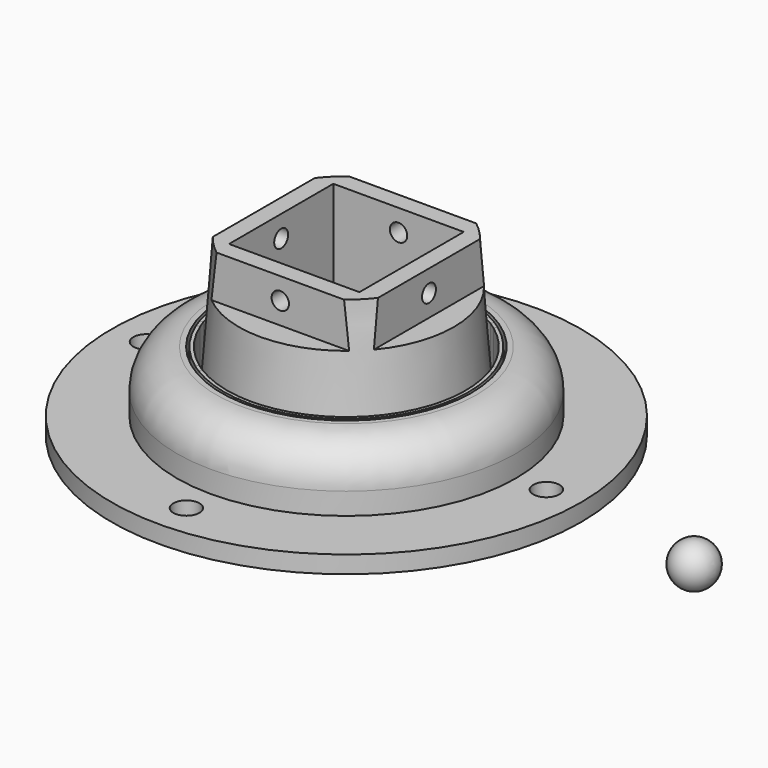
from build123d import *
from build123d import SkipClean  # not in build123d's __all__

# Parameters (mm, degrees)
F3_W           = 38.1
F3_H           = 38.1
F4_DEPTH       = 56.135
F5_DEPTH       = 12.7
F6_R           = 3.81
F7_DEPTH       = 10.415
F14_DEPTH      = 22.86
F15_R          = 6.35
F16_DEPTH      = 101.3661944055
F17_COUNT      = 10
F18_R          = 2.54
F19_DEPTH      = 68.581
F19_DEPTH_BACK = 68.581
F20_R          = 2.54
F21_DEPTH      = 107.951
F21_DEPTH_BACK = 68.581


with BuildPart() as f1:
    # F0 (on Front) → F1 (revolve)
    with BuildSketch(Plane.XZ):
        with BuildLine():
            Line((38.1, 4.445), (38.1, 0))
            Line((38.1, 0), (49.53, 0))
            Line((49.53, 0), (68.58, 0))
            Line((68.58, 0), (68.58, 5.08))
            Line((68.58, 5.08), (49.53, 5.08))
            Line((49.53, 5.08), (49.53, 11.43))
            ThreePointArc((49.53, 11.43), (46.182230509, 19.512230509), (38.1, 22.86))
            Line((38.1, 22.86), (38.1, 18.415))
            ThreePointArc((38.1, 18.415), (43.0391408666, 16.3691408666), (45.085, 11.43))
            ThreePointArc((45.085, 11.43), (43.0391408666, 6.4908591334), (38.1, 4.445))
        make_face()
        with BuildLine():
            Line((36.576, 0), (38.1, 0))
            Line((38.1, 0), (38.1, 4.445))
            ThreePointArc((38.1, 4.445), (37.3333686161, 4.4871978769), (36.576, 4.6132816546))
            Line((36.576, 4.6132816546), (36.576, 0))
        make_face()
        with BuildLine():
            ThreePointArc((36.576, 18.2467183454), (37.3333686161, 18.3728021231), (38.1, 18.415))
            Line((38.1, 18.415), (38.1, 22.86))
            Line((38.1, 22.86), (36.576, 22.86))
            Line((36.576, 22.86), (36.576, 18.2467183454))
        make_face()
    revolve(axis=Axis((0, 0, 43.4834131303), (0, 0, 1)))

    # F6 (on face) → F7 (cut, through all)
    with BuildSketch(Plane.XY.offset(5.08)):
        with Locations((0, 58.42)):
            Circle(F6_R)
        with Locations((58.42, 0)):
            Circle(F6_R)
        with Locations((0, -58.42)):
            Circle(F6_R)
        with Locations((-58.42, 0)):
            Circle(F6_R)
    extrude(amount=-F7_DEPTH, mode=Mode.SUBTRACT)


with BuildPart() as f2:
    # F0 (on Front) → F2 (revolve)
    with BuildSketch(Plane.XZ):
        with BuildLine():
            Line((34.29, 0), (34.29, 5.5755892696))
            ThreePointArc((34.29, 5.5755892696), (31.1641540477, 10.6027963216), (33.02, 16.2241448664))
            Line((33.02, 16.2241448664), (30.48, 50.8))
            Line((30.48, 50.8), (0, 50.8))
            Line((0, 50.8), (0, 0))
            Line((0, 0), (34.29, 0))
        make_face()
        Polygon((34.29, -0.254), (34.29, 0), (0, 0), (0, -5.334), (49.53, -5.334), (49.53, -0.254), align=None)
    revolve(axis=Axis((0, 0, 43.4834131303), (0, 0, 1)))

    # F3 (on face) → F4 (cut, through all)
    with BuildSketch(Plane.XY.offset(50.8)):
        Rectangle(F3_W, F3_H)
    extrude(amount=-F4_DEPTH, mode=Mode.SUBTRACT)

    # F3 (on face) → F5 (cut)
    with BuildSketch(Plane.XY.offset(50.8)):
        with BuildLine():
            Line((18.6218554392, 24.13), (22.5402639736, 24.13))
            ThreePointArc((22.5402639736, 24.13), (0, 33.02), (-22.5402639736, 24.13))
            Line((-22.5402639736, 24.13), (-18.6218554392, 24.13))
            ThreePointArc((-18.6218554392, 24.13), (0, 30.48), (18.6218554392, 24.13))
        make_face()
        with BuildLine():
            ThreePointArc((24.13, -22.5402639736), (30.717202021, -12.115027858), (33.02, 0))
            ThreePointArc((33.02, 0), (30.717202021, 12.115027858), (24.13, 22.5402639736))
            Line((24.13, 22.5402639736), (24.13, 18.6218554392))
            ThreePointArc((24.13, 18.6218554392), (28.8488543967, 9.8373776994), (30.48, 0))
            ThreePointArc((30.48, 0), (28.8488543967, -9.8373776994), (24.13, -18.6218554392))
            Line((24.13, -18.6218554392), (24.13, -22.5402639736))
        make_face()
        with BuildLine():
            ThreePointArc((-22.5402639736, -24.13), (0, -33.02), (22.5402639736, -24.13))
            Line((22.5402639736, -24.13), (18.6218554392, -24.13))
            ThreePointArc((18.6218554392, -24.13), (0, -30.48), (-18.6218554392, -24.13))
            Line((-18.6218554392, -24.13), (-22.5402639736, -24.13))
        make_face()
        with BuildLine():
            Line((-24.13, 18.6218554392), (-24.13, 22.5402639736))
            ThreePointArc((-24.13, 22.5402639736), (-33.02, 0), (-24.13, -22.5402639736))
            Line((-24.13, -22.5402639736), (-24.13, -18.6218554392))
            ThreePointArc((-24.13, -18.6218554392), (-30.48, 0), (-24.13, 18.6218554392))
        make_face()
        with BuildLine():
            Line((-18.6218554392, 24.13), (18.6218554392, 24.13))
            ThreePointArc((18.6218554392, 24.13), (0, 30.48), (-18.6218554392, 24.13))
        make_face()
        with BuildLine():
            ThreePointArc((30.48, 0), (28.8488543967, 9.8373776994), (24.13, 18.6218554392))
            Line((24.13, 18.6218554392), (24.13, -18.6218554392))
            ThreePointArc((24.13, -18.6218554392), (28.8488543967, -9.8373776994), (30.48, 0))
        make_face()
        with BuildLine():
            ThreePointArc((-18.6218554392, -24.13), (0, -30.48), (18.6218554392, -24.13))
            Line((18.6218554392, -24.13), (-18.6218554392, -24.13))
        make_face()
        with BuildLine():
            Line((-24.13, -18.6218554392), (-24.13, 18.6218554392))
            ThreePointArc((-24.13, 18.6218554392), (-30.48, 0), (-24.13, -18.6218554392))
        make_face()
    extrude(amount=-F5_DEPTH, mode=Mode.SUBTRACT)

    # F18 (on Front) → F19 (cut, two sides)
    with BuildSketch(Plane.XZ) as f19_sk:
        with Locations((0, 44.45)):
            Circle(F18_R)
    extrude(amount=-F19_DEPTH, mode=Mode.SUBTRACT)
    extrude(f19_sk.sketch, amount=F19_DEPTH_BACK, mode=Mode.SUBTRACT)

    # F20 (on Right) → F21 (cut, two sides)
    with BuildSketch(Plane.YZ) as f21_sk:
        with Locations((0, 44.45)):
            Circle(F20_R)
    extrude(amount=F21_DEPTH, mode=Mode.SUBTRACT)
    extrude(f21_sk.sketch, amount=-F21_DEPTH_BACK, mode=Mode.SUBTRACT)


with BuildPart() as f9:
    # F8 (on Front) → F9 (revolve)
    with BuildSketch(Plane.XZ):
        with BuildLine():
            Line((101.6, 6.35), (101.6, -6.35))
            ThreePointArc((101.6, -6.35), (107.95, 0), (101.6, 6.35))
        make_face()
    revolve(axis=Axis((101.6, 0, 3.8127312437), (0, 0, 1)))


with BuildPart() as f14:
    # F13 (on face) → F14 (new body, through all)
    with BuildSketch(Plane.XY.offset(22.86)):
        with BuildLine():
            Line((0, -34.798), (0, -35.814))
            ThreePointArc((0, -35.814), (12.2491094131, -33.6541515208), (23.0207954533, -27.4351156859))
            Line((23.0207954533, -27.4351156859), (22.3677232419, -26.6568145317))
            ThreePointArc((22.3677232419, -26.6568145317), (11.9016169474, -32.6994238181), (0, -34.798))
        make_face()
    extrude(amount=-F14_DEPTH)

    # F15 (on line) → F16 (cut, through all)
    with BuildSketch(Plane(origin=(0, 0, 0), x_dir=(-0.9396926208, -0.3420201433, 0), z_dir=(-0.3420201433, 0.9396926208, 0))):
        with Locations((0, 11.43)):
            Circle(F15_R)
    extrude(amount=-F16_DEPTH, mode=Mode.SUBTRACT)

    # F17: F14 ×10 about axis
    f17_axis = Axis((0, 0, 43.4834131303), (0, 0, 1))


with BuildPart() as f14_1:
    add(f14.part, clean=False)
    with SkipClean():  # cleaning this boolean's faces spoils the solid; the shape is the same uncleaned
        for i in range(1, F17_COUNT):
            add(f14.part.rotate(f17_axis, i * 360 / F17_COUNT), clean=False)


solid = Compound([f1.part, f2.part, f9.part, f14_1.part])
